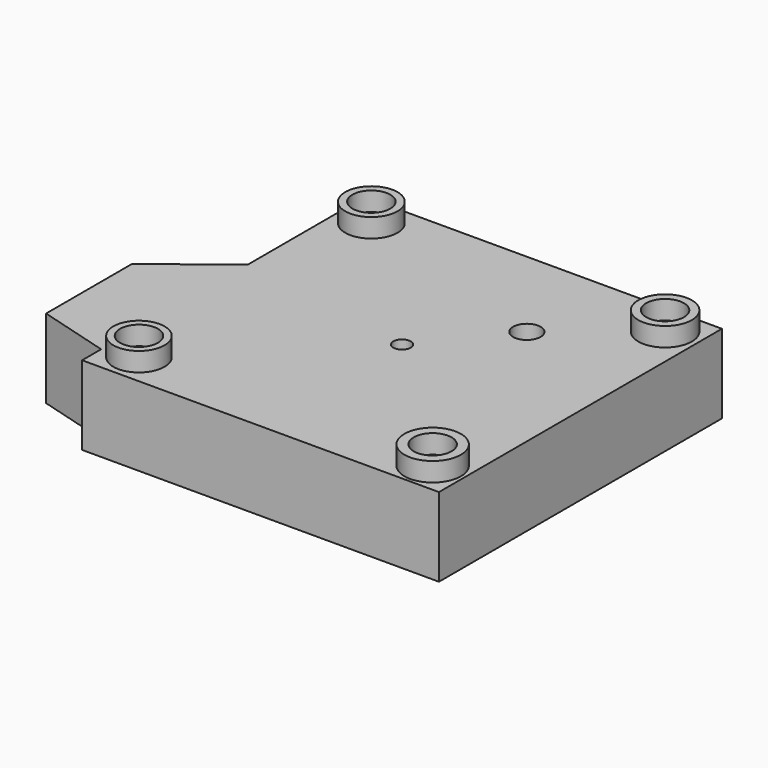
from build123d import *

# Parameters (mm, degrees)
F0_R           = 8.1165547555
F0_R_2         = 8.9540708035
F0_R_3         = 8.2604689148
F0_R_4         = 8.4855933961
F1_DEPTH       = 25
F0_R_5         = 6
F2_DEPTH       = 31
F3_R           = 4.3558335705
F4_DEPTH       = 25
F5_D           = 5.5
F5_CSINK_D     = 11.2
F5_CSINK_ANGLE = 90


with BuildPart() as f1:
    # F0 (on Top) → F1 (new body)
    with BuildSketch(Plane.XY):
        Polygon((-56.5, -56), (56.5, -56), (56.5, 56), (-56.5, 56), (-56.5, 9.6476091864), (-56.5, -48.4666682311), align=None)
        with Locations((-46.5, -46)):
            Circle(F0_R, mode=Mode.SUBTRACT)
        with Locations((46.5, -46)):
            Circle(F0_R_2, mode=Mode.SUBTRACT)
        with Locations((-46.5, 46)):
            Circle(F0_R_3, mode=Mode.SUBTRACT)
        with Locations((46.5, 46)):
            Circle(F0_R_4, mode=Mode.SUBTRACT)
        Polygon((-79.0999777075, -42.0095233626), (-56.5, -48.4666682311), (-56.5, 9.6476091864), (-79.0999777075, -8.1095304023), align=None)
    extrude(amount=F1_DEPTH)

    # F0 (on Top) → F2 (join)
    with BuildSketch(Plane.XY):
        with Locations((-46.5, -46)):
            Circle(F0_R)
        with Locations((-46.5, -46)):
            Circle(F0_R_5, mode=Mode.SUBTRACT)
        with Locations((46.5, -46)):
            Circle(F0_R_2)
        with Locations((46.5, -46)):
            Circle(F0_R_5, mode=Mode.SUBTRACT)
        with Locations((46.5, 46)):
            Circle(F0_R_4)
        with Locations((46.5, 46)):
            Circle(F0_R_5, mode=Mode.SUBTRACT)
        with Locations((-46.5, 46)):
            Circle(F0_R_3)
        with Locations((-46.5, 46)):
            Circle(F0_R_5, mode=Mode.SUBTRACT)
    extrude(amount=F2_DEPTH)

    # F3 (on Top) → F4 (cut, through all)
    with BuildSketch(Plane.XY):
        with Locations((19.8767594993, 24.5702005923)):
            Circle(F3_R)
    extrude(amount=F4_DEPTH, mode=Mode.SUBTRACT)

    # F5 (through all)
    with Locations(Plane(origin=(0, 0, 0), x_dir=(1, 0, 0), z_dir=(0, 0, -1))):
        with Locations((0, 0)):
            CounterSinkHole(F5_D / 2, F5_CSINK_D / 2, counter_sink_angle=F5_CSINK_ANGLE)


with BuildPart() as f1b:
    # F0 (on Top) → F1, piece 2 (new body)
    with BuildSketch(Plane.XY):
        with Locations((-46.5, 46)):
            Circle(F0_R_5)
    extrude(amount=F1_DEPTH)


with BuildPart() as f1c:
    # F0 (on Top) → F1, piece 3 (new body)
    with BuildSketch(Plane.XY):
        with Locations((46.5, 46)):
            Circle(F0_R_5)
    extrude(amount=F1_DEPTH)


with BuildPart() as f1d:
    # F0 (on Top) → F1, piece 4 (new body)
    with BuildSketch(Plane.XY):
        with Locations((46.5, -46)):
            Circle(F0_R_5)
    extrude(amount=F1_DEPTH)


with BuildPart() as f1e:
    # F0 (on Top) → F1, piece 5 (new body)
    with BuildSketch(Plane.XY):
        with Locations((-46.5, -46)):
            Circle(F0_R_5)
    extrude(amount=F1_DEPTH)


solid = Compound([f1.part, f1b.part, f1c.part, f1d.part, f1e.part])
